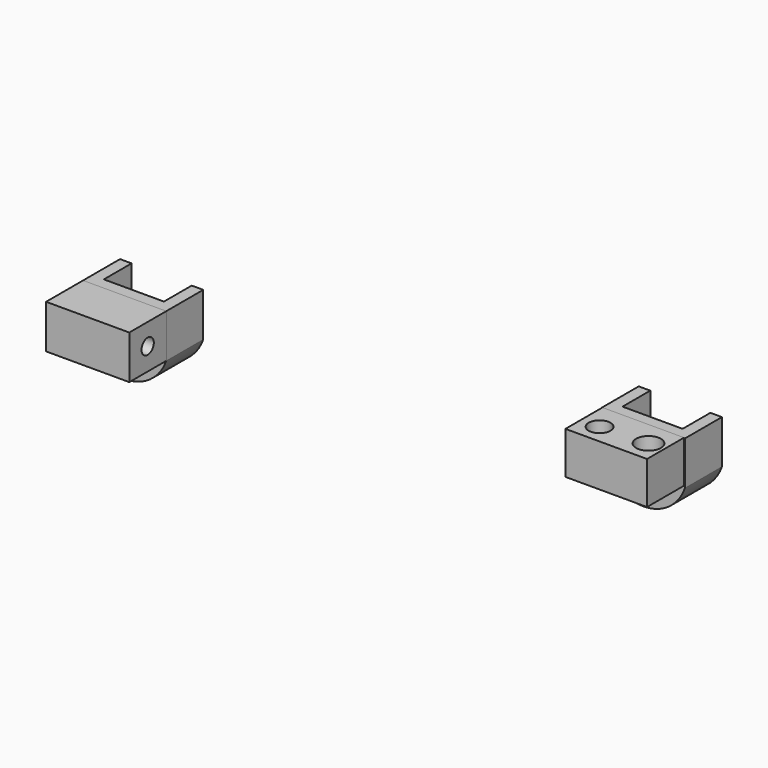
from build123d import *

# Parameters (mm, degrees)
F0_W     = 18
F0_H     = 9.451737664
F1_DEPTH = 10
F2_T     = -2.5
F2_2_T   = -2.5
F3_W     = 18
F3_H     = 9.451737664
F4_DEPTH = 10
F3_W_2   = 17.6508575678
F3_H_2   = 9.1523528099
F5_R     = 2.6878293193
F5_R_2   = 2.3544087044
F6_DEPTH = 25
F7_R     = 1.66
F8_DEPTH = 25


with BuildPart() as f1:
    # F0 (on Front) → F1 (new body)
    with BuildSketch(Plane.XZ):
        with Locations((-61.3145157695, 30.7863325212)):
            Rectangle(F0_W, F0_H)
        with BuildLine():
            Line((-52.3145157695, 26.0604636891), (-70.3145157695, 26.0604636891))
            ThreePointArc((-70.3145157695, 26.0604636891), (-61.3145157695, 19.6358036407), (-52.3145157695, 26.0604636891))
        make_face()
    extrude(amount=F1_DEPTH)

    # F2
    f2_openings = [f1.faces().sort_by_distance(p)[0] for p in [
        (-61.314516, -5, 35.512201),
        (-61.314516, 0, 28.335197),
    ]]
    offset(amount=F2_T, openings=f2_openings)


with BuildPart() as f1b:
    # F0 (on Front) → F1, piece 2 (new body)
    with BuildSketch(Plane.XZ):
        with Locations((50.8881695569, 43.0416602246)):
            Rectangle(F0_W, F0_H)
        with BuildLine():
            Line((59.8881695569, 38.3157913926), (41.8881695569, 38.3157913926))
            ThreePointArc((41.8881695569, 38.3157913926), (50.8881695569, 31.8911313442), (59.8881695569, 38.3157913926))
        make_face()
    extrude(amount=F1_DEPTH)

    # F2#2
    f2_2_openings = [f1b.faces().sort_by_distance(p)[0] for p in [
        (50.88817, 0, 40.590525),
        (50.88817, -5, 47.767529),
    ]]
    offset(amount=F2_2_T, openings=f2_2_openings)

    # F3 (on face) → F4, piece 2 (join)
    with BuildSketch(Plane.XZ.offset(10)):
        with Locations((50.8615411818, 43.2734750211)):
            Rectangle(F3_W_2, F3_H_2)
    extrude(amount=F4_DEPTH)

    # F5 (on face) → F6 (cut)
    with BuildSketch(Plane.XY.offset(47.8496514261)):
        with Locations((56.3105680048, -15.3786037117)):
            Circle(F5_R)
        with Locations((46.058550477, -15.7981198281)):
            Circle(F5_R_2)
    extrude(amount=-F6_DEPTH, mode=Mode.SUBTRACT)


with BuildPart() as f4:
    # F3 (on face) → F4 (new body)
    with BuildSketch(Plane.XZ.offset(10)):
        with Locations((-61.3145157695, 30.7863325212)):
            Rectangle(F3_W, F3_H)
    extrude(amount=F4_DEPTH)

    # F7 (on face) → F8 (cut)
    with BuildSketch(Plane(origin=(-70.3145157695, 0, 0), x_dir=(0, -1, 0), z_dir=(-1, 0, 0))):
        with Locations((15.0299780071, 30.8788195252)):
            Circle(F7_R)
    extrude(amount=-F8_DEPTH, mode=Mode.SUBTRACT)


solid = Compound([f1.part, f1b.part, f4.part])
